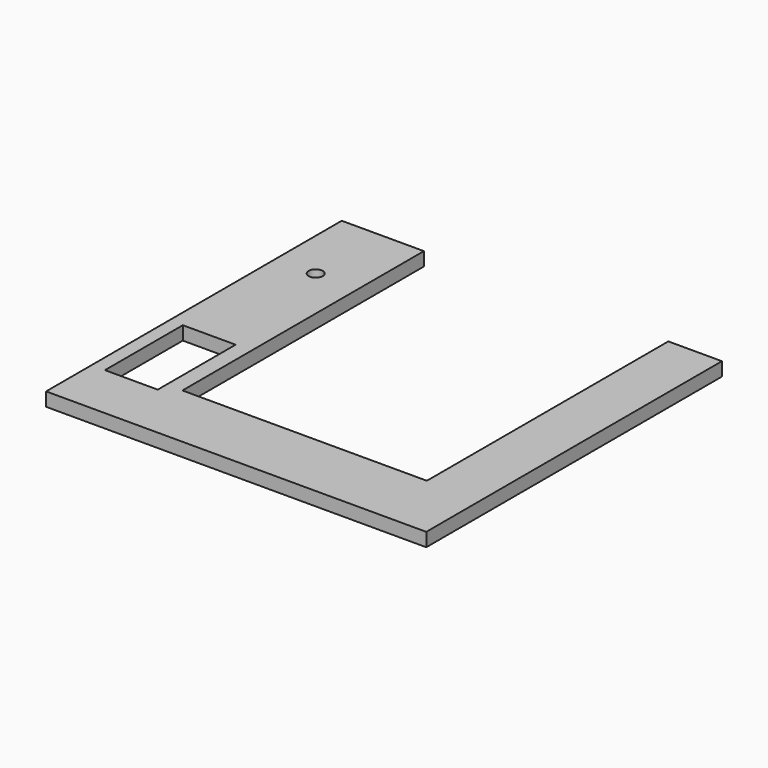
from build123d import *

# Parameters (mm, degrees)
F0_W     = 12.3444
F0_H     = 22.7584
F0_R     = 1.651
F1_DEPTH = 3.175


# Not quite as in the source:
# - a length typed as a fraction of an inch, garbled in the dataset ("3 / 203.2 mm" for 3/8 in), is restored


with BuildPart() as f1:
    # F0 (on Top) → F1 (new body)
    with BuildSketch(Plane.XY):
        Polygon((0, 86.4107935882), (0, 0), (19.2153378795, 0), (88.9, 0), (88.9, 15.8380966835), (88.9, 86.4107935882), (76.3653378795, 86.4107935882), (76.3653378795, 15.8380966835), (19.2153378795, 15.8380966835), (19.2153378795, 86.4107935882), align=None)
        with Locations((9.3165273066, 24.6552514774)):
            Rectangle(F0_W, F0_H, mode=Mode.SUBTRACT)
        with Locations((9.3165273066, 67.1494514774)):
            Circle(F0_R, mode=Mode.SUBTRACT)
    extrude(amount=F1_DEPTH)


solid = f1.part
